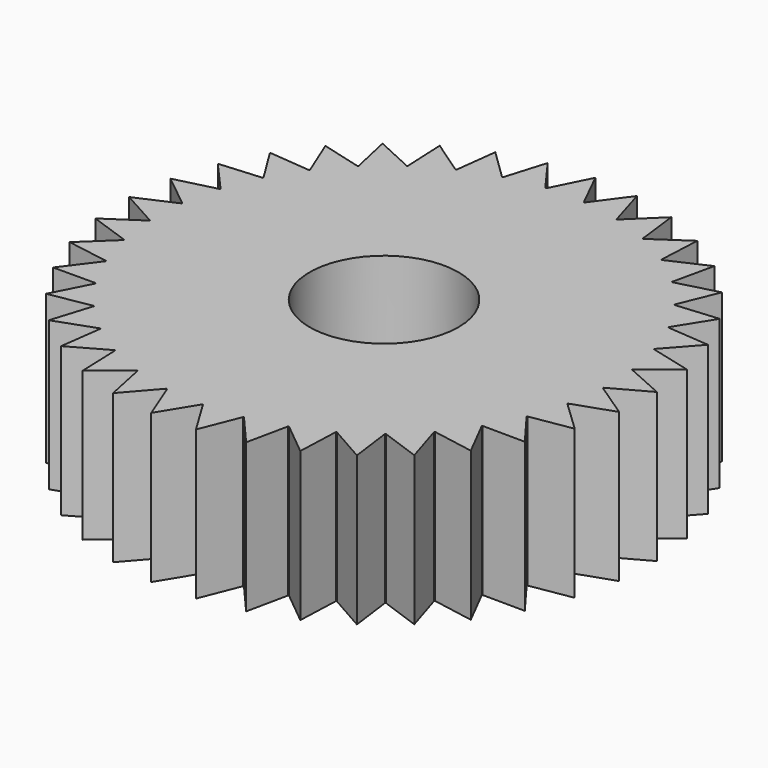
from build123d import *

# Parameters (mm, degrees)
F0_R     = 2.5
F1_DEPTH = 5


# Not quite as in the source:
# - a feature names something its author has since deleted; it is built from what else it names


with BuildPart() as f1:
    # F0 (on Top) → F1 (new body)
    with BuildSketch(Plane.XY):
        with BuildLine():
            ThreePointArc((0.6328035034, 7.5936789322), (-0.0023111215, 7.6199996495), (-0.6374096636, 7.5932936807))
            ThreePointArc((-0.6374096636, 7.5932936807), (-0.6485239105, 7.5923525167), (-0.6596367677, 7.5913950849))
            ThreePointArc((-0.6596367677, 7.5913950849), (-1.2900640698, 7.51000231), (-1.9115139669, 7.3763483076))
            ThreePointArc((-1.9115139669, 7.3763483076), (-1.9223092879, 7.3735423645), (-1.9331004901, 7.3707206225))
            ThreePointArc((-1.9331004901, 7.3707206225), (-2.5407042235, 7.1839558774), (-3.1306274935, 6.9471988237))
            ThreePointArc((-3.1306274935, 6.9471988237), (-3.140793327, 6.9426088236), (-3.1509524309, 6.9380039477))
            ThreePointArc((-3.1509524309, 6.9380039477), (-3.7182529426, 6.651240114), (-4.2596785672, 6.3181910785))
            ThreePointArc((-4.2596785672, 6.3181910785), (-4.2689224606, 6.3119490671), (-4.2781572072, 6.3056935313))
            ThreePointArc((-4.2781572072, 6.3056935313), (-4.7888342944, 5.9271802825), (-5.266186444, 5.5074204794))
            ThreePointArc((-5.266186444, 5.5074204794), (-5.2742424674, 5.4997060281), (-5.2822871898, 5.4919797928))
            ThreePointArc((-5.2822871898, 5.4919797928), (-5.7216496025, 5.0326062658), (-6.1211957249, 4.5382114205))
            ThreePointArc((-6.1211957249, 4.5382114205), (-6.1278321211, 4.52924646), (-6.1344553875, 4.5202717948))
            ThreePointArc((-6.1344553875, 4.5202717948), (-6.4898634689, 3.9932533296), (-6.8001093497, 3.4384462817))
            ThreePointArc((-6.8001093497, 3.4384462817), (-6.8051352017, 3.4284887176), (-6.8101464726, 3.4185238073))
            ThreePointArc((-6.8101464726, 3.4185238073), (-7.0713757794, 2.8390217657), (-7.2833962094, 2.2397633037))
            ThreePointArc((-7.2833962094, 2.2397633037), (-7.2866669326, 2.229099597), (-7.289922043, 2.218431114))
            ThreePointArc((-7.289922043, 2.218431114), (-7.4494574836, 1.6031167146), (-7.557153021, 0.9766464135))
            ThreePointArc((-7.557153021, 0.9766464135), (-7.5585745227, 0.9655833395), (-7.5599798288, 0.9545181966))
            ThreePointArc((-7.5599798288, 0.9545181966), (-7.6132318591, 0.3210929144), (-7.6135042995, -0.314566816))
            ThreePointArc((-7.6135042995, -0.314566816), (-7.6130356855, -0.3257109926), (-7.6125507594, -0.3368544714))
            ThreePointArc((-7.6125507594, -0.3368544714), (-7.5579874154, -0.9701681444), (-7.4508289211, -1.5967305308))
            ThreePointArc((-7.4508289211, -1.5967305308), (-7.4484836728, -1.6076352125), (-7.4461224648, -1.6185364495))
            ThreePointArc((-7.4461224648, -1.6185364495), (-7.2853134346, -2.233519232), (-7.0738067604, -2.8329592155))
            ThreePointArc((-7.0738067604, -2.8329592155), (-7.0696523462, -2.8433106943), (-7.0654827841, -2.8536560809))
            ThreePointArc((-7.0654827841, -2.8536560809), (-6.8030542506, -3.4326160379), (-6.4932840584, -3.9876888214))
            ThreePointArc((-6.4932840584, -3.9876888214), (-6.4874399932, -3.9971893043), (-6.4815820277, -4.0066812225))
            ThreePointArc((-6.4815820277, -4.0066812225), (-6.1250835821, -4.5329627301), (-5.7259613964, -5.0276998804))
            ThreePointArc((-5.7259613964, -5.0276998804), (-5.7185958034, -5.0360760556), (-5.7112179573, -5.0444414402))
            ThreePointArc((-5.7112179573, -5.0444414402), (-5.2709054108, -5.5029043377), (-4.7939132502, -5.9230731677))
            ThreePointArc((-4.7939132502, -5.9230731677), (-4.785238024, -5.930084068), (-4.7765525447, -5.9370822621))
            ThreePointArc((-4.7765525447, -5.9370822621), (-4.2650928876, -6.3145374066), (-3.7239529481, -6.648050424))
            ThreePointArc((-3.7239529481, -6.648050424), (-3.7142176592, -6.6534943586), (-3.7044744121, -6.658924037))
            ThreePointArc((-3.7044744121, -6.658924037), (-3.1365814075, -6.9445127312), (-2.5468612998, -7.1817753738))
            ThreePointArc((-2.5468612998, -7.1817753738), (-2.5363460148, -7.1854957305), (-2.5258252953, -7.1892006911))
            ThreePointArc((-2.5258252953, -7.1892006911), (-1.917836191, -7.3747070684), (-1.296501089, -7.5088937219))
            ThreePointArc((-1.296501089, -7.5088937219), (-1.2855083135, -7.5107834728), (-1.2745127836, -7.5126571308))
            ThreePointArc((-1.2745127836, -7.5126571308), (-0.6439183191, -7.5927445103), (-0.0088429024, -7.619994869))
            ThreePointArc((-0.0088429024, -7.619994869), (0.0023111215, -7.6199996495), (0.0134651405, -7.619988103))
            ThreePointArc((0.0134651405, -7.619988103), (0.6485239105, -7.5923525167), (1.2790696784, -7.5118826374))
            ThreePointArc((1.2790696784, -7.5118826374), (1.2900640698, -7.51000231), (1.3010556969, -7.5081058912))
            ThreePointArc((1.3010556969, -7.5081058912), (1.9223092879, -7.3735423645), (2.5301857534, -7.1876672192))
            ThreePointArc((2.5301857534, -7.1876672192), (2.5407042235, -7.1839558774), (2.5512172498, -7.1802291429))
            ThreePointArc((2.5512172498, -7.1802291429), (3.140793327, -6.9426088236), (3.7085129909, -6.6566757016))
            ThreePointArc((3.7085129909, -6.6566757016), (3.7182529426, -6.651240114), (3.7279849274, -6.6457902751))
            ThreePointArc((3.7279849274, -6.6457902751), (4.2689224606, -6.3119490671), (4.7801530617, -5.9341837439))
            ThreePointArc((4.7801530617, -5.9341837439), (4.7888342944, -5.9271802825), (4.7975052662, -5.9201641211))
            ThreePointArc((4.7975052662, -5.9201641211), (5.2742424674, -5.4997060281), (5.7142768322, -5.0409761242))
            ThreePointArc((5.7142768322, -5.0409761242), (5.7216496025, -5.0326062658), (5.7290101132, -5.0242256241))
            ThreePointArc((5.7290101132, -5.0242256241), (6.1278321211, -4.52924646), (6.4840112622, -4.0027487995))
            ThreePointArc((6.4840112622, -4.0027487995), (6.4898634689, -3.9932533296), (6.4957017701, -3.9837493036))
            ThreePointArc((6.4957017701, -3.9837493036), (6.8051352017, -3.4284887176), (7.0672124935, -2.8493696796))
            ThreePointArc((7.0672124935, -2.8493696796), (7.0713757794, -2.8390217657), (7.0755239138, -2.8286677687))
            ThreePointArc((7.0755239138, -2.8286677687), (7.2866669326, -2.229099597), (7.4471028887, -1.6140193819))
            ThreePointArc((7.4471028887, -1.6140193819), (7.4494574836, -1.6031167146), (7.4517961168, -1.5922106123))
            ThreePointArc((7.4517961168, -1.5922106123), (7.5585745227, -0.9655833395), (7.6127536927, -0.3322366852))
            ThreePointArc((7.6127536927, -0.3322366852), (7.6132318591, -0.3210929144), (7.613693713, -0.3099484555))
            ThreePointArc((7.613693713, -0.3099484555), (7.6184232651, -0.1550063017), (7.62, 0))
            ThreePointArc((7.62, 0), (7.6048347675, 0.4805082297), (7.5593994334, 0.959103856))
            ThreePointArc((7.5593994334, 0.959103856), (7.5579874154, 0.9701681444), (7.5565592033, 0.981230354))
            ThreePointArc((7.5565592033, 0.981230354), (7.4484836728, 1.6076352125), (7.2885750158, 2.2228527255))
            ThreePointArc((7.2885750158, 2.2228527255), (7.2853134346, 2.233519232), (7.2820362435, 2.2441809528))
            ThreePointArc((7.2820362435, 2.2441809528), (7.0696523462, 2.8433106943), (6.8080715652, 3.4226541693))
            ThreePointArc((6.8080715652, 3.4226541693), (6.8030542506, 3.4326160379), (6.7980223593, 3.4425705516))
            ThreePointArc((6.7980223593, 3.4425705516), (6.4874399932, 3.9971893043), (6.1317122912, 4.5239920842))
            ThreePointArc((6.1317122912, 4.5239920842), (6.1250835821, 4.5329627301), (6.118441749, 4.5419236634))
            ThreePointArc((6.118441749, 4.5419236634), (5.7185958034, 5.0360760556), (5.2789548185, 5.4951829837))
            ThreePointArc((5.2789548185, 5.4951829837), (5.2709054108, 5.5029043377), (5.2628447094, 5.5106139009))
            ThreePointArc((5.2628447094, 5.5106139009), (4.785238024, 5.930084068), (4.2743314271, 6.3082874738))
            ThreePointArc((4.2743314271, 6.3082874738), (4.2650928876, 6.3145374066), (4.2558452095, 6.3207738096))
            ThreePointArc((4.2558452095, 6.3207738096), (3.7142176592, 6.6534943586), (3.1467433027, 6.9399140187))
            ThreePointArc((3.1467433027, 6.9399140187), (3.1365814075, 6.9445127312), (3.1264127916, 6.9490965641))
            ThreePointArc((3.1264127916, 6.9490965641), (2.5363460148, 7.1854957305), (1.9286291028, 7.3718918728))
            ThreePointArc((1.9286291028, 7.3718918728), (1.917836191, 7.3747070684), (1.9070391699, 7.3775064625))
            ThreePointArc((1.9070391699, 7.3775064625), (1.2855083135, 7.5107834728), (0.6550317551, 7.5917938196))
            ThreePointArc((0.6550317551, 7.5917938196), (0.6439183191, 7.5927445103), (0.6328035034, 7.5936789322))
        make_face()
        Circle(F0_R, mode=Mode.SUBTRACT)
        with BuildLine():
            ThreePointArc((-6.1211957249, 4.5382114205), (-5.7216496025, 5.0326062658), (-5.2822871898, 5.4919797928))
            Line((-5.2822871898, 5.4919797928), (-6.6584633476, 5.8601847965))
            Line((-6.6584633476, 5.8601847965), (-6.1211957249, 4.5382114205))
        make_face()
        with BuildLine():
            ThreePointArc((-5.266186444, 5.5074204794), (-4.7888342944, 5.9271802825), (-4.2781572072, 6.3056935313))
            Line((-4.2781572072, 6.3056935313), (-5.572311376, 6.9011771408))
            Line((-5.572311376, 6.9011771408), (-5.266186444, 5.5074204794))
        make_face()
        with BuildLine():
            ThreePointArc((-4.2596785672, 6.3181910785), (-3.7182529426, 6.651240114), (-3.1509524309, 6.9380039477))
            Line((-3.1509524309, 6.9380039477), (-4.3258541516, 7.7436351837))
            Line((-4.3258541516, 7.7436351837), (-4.2596785672, 6.3181910785))
        make_face()
        with BuildLine():
            ThreePointArc((-3.1306274935, 6.9471988237), (-2.5407042235, 7.1839558774), (-1.9331004901, 7.3707206225))
            Line((-1.9331004901, 7.3707206225), (-2.9549499794, 8.3633229412))
            Line((-2.9549499794, 8.3633229412), (-3.1306274935, 6.9471988237))
        make_face()
        with BuildLine():
            ThreePointArc((-1.9115139669, 7.3763483076), (-1.2900640698, 7.51000231), (-0.6596367677, 7.5913950849))
            Line((-0.6596367677, 7.5913950849), (-1.4990372763, 8.7424131248))
            Line((-1.4990372763, 8.7424131248), (-1.9115139669, 7.3763483076))
        make_face()
        with BuildLine():
            Line((1.4990372763, 8.7424131248), (0.6550317551, 7.5917938196))
            ThreePointArc((0.6550317551, 7.5917938196), (1.2855083135, 7.5107834728), (1.9070391699, 7.3775064625))
            Line((1.9070391699, 7.3775064625), (1.4990372763, 8.7424131248))
        make_face()
        with BuildLine():
            Line((2.9549499794, 8.3633229412), (1.9286291028, 7.3718918728))
            ThreePointArc((1.9286291028, 7.3718918728), (2.5363460148, 7.1854957305), (3.1264127916, 6.9490965641))
            Line((3.1264127916, 6.9490965641), (2.9549499794, 8.3633229412))
        make_face()
        with BuildLine():
            Line((4.3258541516, 7.7436351837), (3.1467433027, 6.9399140187))
            ThreePointArc((3.1467433027, 6.9399140187), (3.7142176592, 6.6534943586), (4.2558452095, 6.3207738096))
            Line((4.2558452095, 6.3207738096), (4.3258541516, 7.7436351837))
        make_face()
        with BuildLine():
            Line((5.572311376, 6.9011771408), (4.2743314271, 6.3082874738))
            ThreePointArc((4.2743314271, 6.3082874738), (4.785238024, 5.930084068), (5.2628447094, 5.5106139009))
            Line((5.2628447094, 5.5106139009), (5.572311376, 6.9011771408))
        make_face()
        with BuildLine():
            Line((6.6584633476, 5.8601847965), (5.2789548185, 5.4951829837))
            ThreePointArc((5.2789548185, 5.4951829837), (5.7185958034, 5.0360760556), (6.118441749, 4.5419236634))
            Line((6.118441749, 4.5419236634), (6.6584633476, 5.8601847965))
        make_face()
        with BuildLine():
            Line((7.5530634517, 4.6506056052), (6.1317122912, 4.5239920842))
            ThreePointArc((6.1317122912, 4.5239920842), (6.4874399932, 3.9971893043), (6.7980223593, 3.4425705516))
            Line((6.7980223593, 3.4425705516), (7.5530634517, 4.6506056052))
        make_face()
        with BuildLine():
            Line((8.2303756721, 3.3072369579), (6.8080715652, 3.4226541693))
            ThreePointArc((6.8080715652, 3.4226541693), (7.0696523462, 2.8433106943), (7.2820362435, 2.2441809528))
            Line((7.2820362435, 2.2441809528), (8.2303756721, 3.3072369579))
        make_face()
        with BuildLine():
            Line((8.6709149695, 1.8687251249), (7.2885750158, 2.2228527255))
            ThreePointArc((7.2885750158, 2.2228527255), (7.4484836728, 1.6076352125), (7.5565592033, 0.981230354))
            Line((7.5565592033, 0.981230354), (8.6709149695, 1.8687251249))
        make_face()
        with BuildLine():
            Line((8.8620078302, 0.3764534723), (7.5593994334, 0.959103856))
            ThreePointArc((7.5593994334, 0.959103856), (7.6048347675, 0.4805082297), (7.62, 0))
            ThreePointArc((7.62, 0), (7.6184232651, -0.1550063017), (7.613693713, -0.3099484555))
            Line((7.613693713, -0.3099484555), (8.8620078302, 0.3764534723))
        make_face()
        with BuildLine():
            Line((8.7981568607, -1.1266480612), (7.6127536927, -0.3322366852))
            ThreePointArc((7.6127536927, -0.3322366852), (7.5585745227, -0.9655833395), (7.4517961168, -1.5922106123))
            Line((7.4517961168, -1.5922106123), (8.7981568607, -1.1266480612))
        make_face()
        with BuildLine():
            Line((8.4811989371, -2.5973379812), (7.4471028887, -1.6140193819))
            ThreePointArc((7.4471028887, -1.6140193819), (7.2866669326, -2.229099597), (7.0755239138, -2.8286677687))
            Line((7.0755239138, -2.8286677687), (8.4811989371, -2.5973379812))
        make_face()
        with BuildLine():
            Line((7.9202523618, -3.9933072165), (7.0672124935, -2.8493696796))
            ThreePointArc((7.0672124935, -2.8493696796), (6.8051352017, -3.4284887176), (6.4957017701, -3.9837493036))
            Line((6.4957017701, -3.9837493036), (7.9202523618, -3.9933072165))
        make_face()
        with BuildLine():
            Line((7.1314545464, -5.2743962738), (6.4840112622, -4.0027487995))
            ThreePointArc((6.4840112622, -4.0027487995), (6.1278321211, -4.52924646), (5.7290101132, -5.0242256241))
            Line((5.7290101132, -5.0242256241), (7.1314545464, -5.2743962738))
        make_face()
        with BuildLine():
            Line((6.1374977678, -6.4037505534), (5.7142768322, -5.0409761242))
            ThreePointArc((5.7142768322, -5.0409761242), (5.2742424674, -5.4997060281), (4.7975052662, -5.9201641211))
            Line((4.7975052662, -5.9201641211), (6.1374977678, -6.4037505534))
        make_face()
        with BuildLine():
            Line((4.966976353, -7.3488805888), (4.7801530617, -5.9341837439))
            ThreePointArc((4.7801530617, -5.9341837439), (4.2689224606, -6.3119490671), (3.7279849274, -6.6457902751))
            Line((3.7279849274, -6.6457902751), (4.966976353, -7.3488805888))
        make_face()
        with BuildLine():
            Line((3.6535640719, -8.0825967097), (3.7085129909, -6.6566757016))
            ThreePointArc((3.7085129909, -6.6566757016), (3.140793327, -6.9426088236), (2.5512172498, -7.1802291429))
            Line((2.5512172498, -7.1802291429), (3.6535640719, -8.0825967097))
        make_face()
        with BuildLine():
            Line((2.2350454045, -8.5837912393), (2.5301857534, -7.1876672192))
            ThreePointArc((2.5301857534, -7.1876672192), (1.9223092879, -7.3735423645), (1.3010556969, -7.5081058912))
            Line((1.3010556969, -7.5081058912), (2.2350454045, -8.5837912393))
        make_face()
        with BuildLine():
            Line((0.7522285501, -8.8380457234), (1.2790696784, -7.5118826374))
            ThreePointArc((1.2790696784, -7.5118826374), (0.6485239105, -7.5923525167), (0.0134651405, -7.619988103))
            Line((0.0134651405, -7.619988103), (0.7522285501, -8.8380457234))
        make_face()
        with BuildLine():
            ThreePointArc((-0.0088429024, -7.619994869), (-0.6439183191, -7.5927445103), (-1.2745127836, -7.5126571308))
            Line((-1.2745127836, -7.5126571308), (-0.7522285501, -8.8380457234))
            Line((-0.7522285501, -8.8380457234), (-0.0088429024, -7.619994869))
        make_face()
        with BuildLine():
            ThreePointArc((-1.296501089, -7.5088937219), (-1.917836191, -7.3747070684), (-2.5258252953, -7.1892006911))
            Line((-2.5258252953, -7.1892006911), (-2.2350454045, -8.5837912393))
            Line((-2.2350454045, -8.5837912393), (-1.296501089, -7.5088937219))
        make_face()
        with BuildLine():
            ThreePointArc((-2.5468612998, -7.1817753738), (-3.1365814075, -6.9445127312), (-3.7044744121, -6.658924037))
            Line((-3.7044744121, -6.658924037), (-3.6535640719, -8.0825967097))
            Line((-3.6535640719, -8.0825967097), (-2.5468612998, -7.1817753738))
        make_face()
        with BuildLine():
            ThreePointArc((-3.7239529481, -6.648050424), (-4.2650928876, -6.3145374066), (-4.7765525447, -5.9370822621))
            Line((-4.7765525447, -5.9370822621), (-4.966976353, -7.3488805888))
            Line((-4.966976353, -7.3488805888), (-3.7239529481, -6.648050424))
        make_face()
        with BuildLine():
            ThreePointArc((-4.7939132502, -5.9230731677), (-5.2709054108, -5.5029043377), (-5.7112179573, -5.0444414402))
            Line((-5.7112179573, -5.0444414402), (-6.1374977678, -6.4037505534))
            Line((-6.1374977678, -6.4037505534), (-4.7939132502, -5.9230731677))
        make_face()
        with BuildLine():
            ThreePointArc((-5.7259613964, -5.0276998804), (-6.1250835821, -4.5329627301), (-6.4815820277, -4.0066812225))
            Line((-6.4815820277, -4.0066812225), (-7.1314545464, -5.2743962738))
            Line((-7.1314545464, -5.2743962738), (-5.7259613964, -5.0276998804))
        make_face()
        with BuildLine():
            ThreePointArc((-6.4932840584, -3.9876888214), (-6.8030542506, -3.4326160379), (-7.0654827841, -2.8536560809))
            Line((-7.0654827841, -2.8536560809), (-7.9202523618, -3.9933072165))
            Line((-7.9202523618, -3.9933072165), (-6.4932840584, -3.9876888214))
        make_face()
        with BuildLine():
            ThreePointArc((-7.0738067604, -2.8329592155), (-7.2853134346, -2.233519232), (-7.4461224648, -1.6185364495))
            Line((-7.4461224648, -1.6185364495), (-8.4811989371, -2.5973379812))
            Line((-8.4811989371, -2.5973379812), (-7.0738067604, -2.8329592155))
        make_face()
        with BuildLine():
            ThreePointArc((-7.4508289211, -1.5967305308), (-7.5579874154, -0.9701681444), (-7.6125507594, -0.3368544714))
            Line((-7.6125507594, -0.3368544714), (-8.7981568607, -1.1266480612))
            Line((-8.7981568607, -1.1266480612), (-7.4508289211, -1.5967305308))
        make_face()
        with BuildLine():
            ThreePointArc((-7.6135042995, -0.314566816), (-7.6132318591, 0.3210929144), (-7.5599798288, 0.9545181966))
            Line((-7.5599798288, 0.9545181966), (-8.8620078302, 0.3764534723))
            Line((-8.8620078302, 0.3764534723), (-7.6135042995, -0.314566816))
        make_face()
        with BuildLine():
            ThreePointArc((-7.557153021, 0.9766464135), (-7.4494574836, 1.6031167146), (-7.289922043, 2.218431114))
            Line((-7.289922043, 2.218431114), (-8.6709149695, 1.8687251249))
            Line((-8.6709149695, 1.8687251249), (-7.557153021, 0.9766464135))
        make_face()
        with BuildLine():
            ThreePointArc((-7.2833962094, 2.2397633037), (-7.0713757794, 2.8390217657), (-6.8101464726, 3.4185238073))
            Line((-6.8101464726, 3.4185238073), (-8.2303756721, 3.3072369579))
            Line((-8.2303756721, 3.3072369579), (-7.2833962094, 2.2397633037))
        make_face()
        with BuildLine():
            ThreePointArc((-6.8001093497, 3.4384462817), (-6.4898634689, 3.9932533296), (-6.1344553875, 4.5202717948))
            Line((-6.1344553875, 4.5202717948), (-7.5530634517, 4.6506056052))
            Line((-7.5530634517, 4.6506056052), (-6.8001093497, 3.4384462817))
        make_face()
        with BuildLine():
            Line((0.6328035034, 7.5936789322), (0, 8.87))
            Line((0, 8.87), (-0.6374096636, 7.5932936807))
            ThreePointArc((-0.6374096636, 7.5932936807), (-0.0023111215, 7.6199996495), (0.6328035034, 7.5936789322))
        make_face()
    extrude(amount=F1_DEPTH)


solid = f1.part
